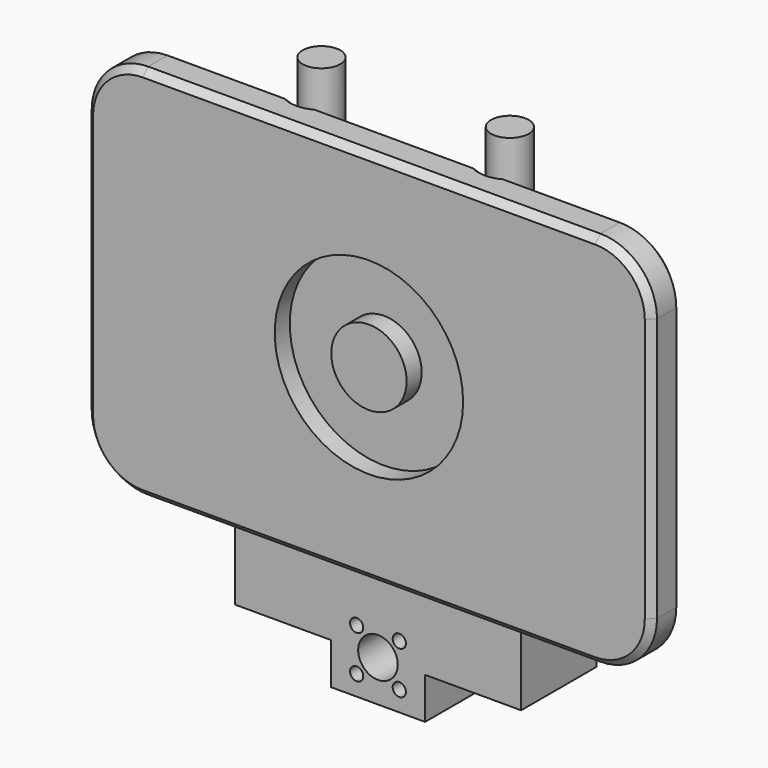
from build123d import *

# Parameters (mm, degrees)
F0_R           = 1.75
F0_R_2         = 5.25
F1_DEPTH       = 25
F2_R           = 1.25
F3_DEPTH       = 19
F2_R_2         = 2.25
F4_DEPTH       = 3.75
F5_R           = 5.2
F6_DEPTH       = 12
F7_R           = 5
F8_DEPTH       = 120
F10_R          = 6.5
F10_R_2        = 5
F11_DEPTH      = 25
F13_W          = 150
F13_H          = 100
F14_DEPTH      = 10
F15_R          = 25
F15_R_2        = 10
F16_DEPTH      = 5
F17_DEPTH      = 55.001
F17_DEPTH_BACK = 83.001
F18_R          = 15
F19_C1_SIZE    = 1.8
F19_C2_SIZE    = 1.8


with BuildPart() as f1:
    # F0 (on Front) → F1 (new body)
    with BuildSketch(Plane.XZ):
        Polygon((38, 11), (38, 30), (-38, 30), (-38, 11), (-12.5, 11), (-12.5, 0), (12.5, 0), (12.5, 11), align=None)
        with Locations((-5.6568542495, 5.3431457505)):
            Circle(F0_R, mode=Mode.SUBTRACT)
        with Locations((5.6568542495, 5.3431457505)):
            Circle(F0_R, mode=Mode.SUBTRACT)
        with Locations((0, 11)):
            Circle(F0_R_2, mode=Mode.SUBTRACT)
        with Locations((-5.6568542495, 16.6568542495)):
            Circle(F0_R, mode=Mode.SUBTRACT)
        with Locations((5.6568542495, 16.6568542495)):
            Circle(F0_R, mode=Mode.SUBTRACT)
    extrude(amount=F1_DEPTH)

    # F2 (on face) → F3 (cut, through all)
    with BuildSketch(Plane.XY.offset(30)):
        with Locations((-32.5, -20.5)):
            Circle(F2_R)
        with Locations((-32.5, -4.5)):
            Circle(F2_R)
        with Locations((-17.5, -4.5)):
            Circle(F2_R)
        with Locations((-17.5, -20.5)):
            Circle(F2_R)
        with Locations((17.5, -4.5)):
            Circle(F2_R)
        with Locations((17.5, -20.5)):
            Circle(F2_R)
        with Locations((32.5, -20.5)):
            Circle(F2_R)
        with Locations((32.5, -4.5)):
            Circle(F2_R)
    extrude(amount=-F3_DEPTH, mode=Mode.SUBTRACT)

    # F2 (on face) → F4 (cut)
    with BuildSketch(Plane.XY.offset(30)):
        with Locations((17.5, -4.5)):
            Circle(F2_R_2)
        with Locations((17.5, -4.5)):
            Circle(F2_R, mode=Mode.SUBTRACT)
        with Locations((17.5, -20.5)):
            Circle(F2_R_2)
        with Locations((17.5, -20.5)):
            Circle(F2_R, mode=Mode.SUBTRACT)
        with Locations((32.5, -20.5)):
            Circle(F2_R_2)
        with Locations((32.5, -20.5)):
            Circle(F2_R, mode=Mode.SUBTRACT)
        with Locations((32.5, -4.5)):
            Circle(F2_R_2)
        with Locations((32.5, -4.5)):
            Circle(F2_R, mode=Mode.SUBTRACT)
        with Locations((-32.5, -4.5)):
            Circle(F2_R_2)
        with Locations((-32.5, -4.5)):
            Circle(F2_R, mode=Mode.SUBTRACT)
        with Locations((-17.5, -4.5)):
            Circle(F2_R_2)
        with Locations((-17.5, -4.5)):
            Circle(F2_R, mode=Mode.SUBTRACT)
        with Locations((-17.5, -20.5)):
            Circle(F2_R_2)
        with Locations((-17.5, -20.5)):
            Circle(F2_R, mode=Mode.SUBTRACT)
        with Locations((-32.5, -20.5)):
            Circle(F2_R_2)
        with Locations((-32.5, -20.5)):
            Circle(F2_R, mode=Mode.SUBTRACT)
    extrude(amount=-F4_DEPTH, mode=Mode.SUBTRACT)

    # F5 (on face) → F6 (cut)
    with BuildSketch(Plane.XY.offset(30)):
        with Locations((-25, -12.5)):
            Circle(F5_R)
        with Locations((25, -12.5)):
            Circle(F5_R)
    extrude(amount=-F6_DEPTH, mode=Mode.SUBTRACT)


with BuildPart() as f8:
    # F7 (on face) → F8 (new body)
    with BuildSketch(Plane.XY.offset(18)):
        with Locations((-25, -12.5)):
            Circle(F7_R)
    extrude(amount=F8_DEPTH)


with BuildPart() as f8b:
    # F7 (on face) → F8, piece 2 (new body)
    with BuildSketch(Plane.XY.offset(18)):
        with Locations((25, -12.5)):
            Circle(F7_R)
    extrude(amount=F8_DEPTH)


with BuildPart() as f11:
    # F10 (on offset) → F11 (new body)
    with BuildSketch(Plane.XY.offset(55)):
        with Locations((25, -12.5)):
            Circle(F10_R)
        with Locations((25, -12.5)):
            Circle(F10_R_2, mode=Mode.SUBTRACT)
    extrude(amount=F11_DEPTH)


with BuildPart() as f11b:
    # F10 (on offset) → F11, piece 2 (new body)
    with BuildSketch(Plane.XY.offset(55)):
        with Locations((-25, -12.5)):
            Circle(F10_R)
        with Locations((-25, -12.5)):
            Circle(F10_R_2, mode=Mode.SUBTRACT)
    extrude(amount=F11_DEPTH)


with BuildPart() as f14:
    # F13 (on offset) → F14 (new body)
    with BuildSketch(Plane.XZ.offset(18)):
        with Locations((0, 80)):
            Rectangle(F13_W, F13_H)
    extrude(amount=F14_DEPTH)

    # F15 (on face) → F16 (cut)
    with BuildSketch(Plane.XZ.offset(28)):
        with Locations((0, 80)):
            Circle(F15_R)
        with Locations((0, 80)):
            Circle(F15_R_2, mode=Mode.SUBTRACT)
    extrude(amount=-F16_DEPTH, mode=Mode.SUBTRACT)

    # F10 (on offset) → F17 (cut, two sides)
    with BuildSketch(Plane.XY.offset(55)) as f17_sk:
        with Locations((25, -12.5)):
            Circle(F10_R)
        with Locations((25, -12.5)):
            Circle(F10_R_2, mode=Mode.SUBTRACT)
        with Locations((-25, -12.5)):
            Circle(F10_R)
        with Locations((-25, -12.5)):
            Circle(F10_R_2, mode=Mode.SUBTRACT)
    extrude(amount=-F17_DEPTH, mode=Mode.SUBTRACT)
    extrude(f17_sk.sketch, amount=F17_DEPTH_BACK, mode=Mode.SUBTRACT)

    # F18
    f18_edges = [f14.edges().sort_by_distance(p)[0] for p in [
        (-75, -23, 130),
        (-75, -23, 30),
        (75, -23, 30),
        (75, -23, 130),
    ]]
    fillet(f18_edges, radius=F18_R)

    # F19: chamfer of 1.8 on 32 edges, made by hand

    # F19_c1
    f19_c1_edges = [f14.edges().sort_by_distance(p)[0] for p in [
        (25, -19, 130),
        (0, -18, 130),
        (-25, -19, 130),
        (-25, -19, 30),
        (0, -18, 30),
        (25, -19, 30),
    ]]
    chamfer(f19_c1_edges, length=F19_C1_SIZE)

    # F19_c2
    f19_c2_edges = [f14.edges().sort_by_distance(p)[0] for p in [
        (45.6080540536, -18, 130),
        (0, -28, 130),
        (-45.6080540536, -18, 130),
        (-70.6066017178, -18, 125.6066017178),
        (-70.6066017178, -28, 125.6066017178),
        (-75, -18, 80),
        (-75, -28, 80),
        (-70.6066017178, -18, 34.3933982822),
        (-70.6066017178, -28, 34.3933982822),
        (-45.6080540536, -18, 30),
        (0, -28, 30),
        (45.6080540536, -18, 30),
        (70.6066017178, -18, 34.3933982822),
        (70.6066017178, -28, 34.3933982822),
        (75, -18, 80),
        (75, -28, 80),
        (70.6066017178, -18, 125.6066017178),
        (70.6066017178, -28, 125.6066017178),
    ]]
    chamfer(f19_c2_edges, length=F19_C2_SIZE)


solid = Compound([f1.part, f8.part, f8b.part, f11.part, f11b.part, f14.part])
